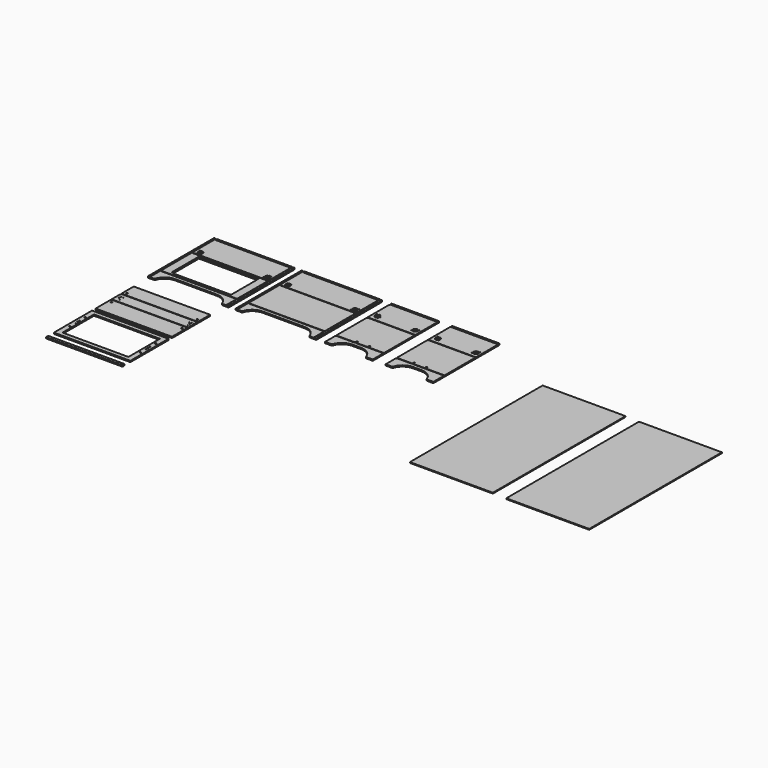
from build123d import *

# Parameters (mm, degrees)
F0_W          = 546.8
F0_H          = 275
F0_W_2        = 10
F0_H_2        = 600
F0_H_3        = 110.9
F0_H_4        = 76
F0_H_5        = 9.1
F0_H_6        = 10
F1_DEPTH      = 9
F0_W_3        = 435
F0_H_7        = 250.55
F0_W_4        = 425
F0_H_8        = 240.55
F0_W_5        = 185
F0_H_9        = 50
F0_W_6        = 345
F0_W_7        = 9.1
F0_H_10       = 17.1
F0_W_8        = 552.8
F0_H_11       = 345
F0_W_9        = 476.8
F0_H_12       = 285
F0_H_13       = 135.9
F0_H_14       = 80
F0_R          = 27.2912012127
F0_H_15       = 20
F2_DEPTH      = 3
F3_R          = 3.3
F3_R_2        = 17.5
F3_R_3        = 6
F3_R_4        = 5
F3_R_5        = 4.25
F3_R_6        = 2.5
F3_R_7        = 1.5
F4_DEPTH      = 16.75
F5_W          = 600
F5_H          = 1200
F6_DEPTH      = 6
F7_T1_DEPTH   = 9
F7_2_T1_DEPTH = 9
F7_3_T1_DEPTH = 9
F7_4_T1_DEPTH = 9
F8_R          = 5
F8_2_R        = 5
F8_3_R        = 5
F8_4_R        = 5


# Not quite as in the source:
# - a fillet or chamfer that OpenCascade refuses, or shapes differently, is made with other operations: its cross-section is extruded or revolved along the edge and cut away or added
# - a feature names something its author has since deleted; it is built from what else it names


with BuildPart() as f1:
    # F0 (on Top) → F1 (new body)
    with BuildSketch(Plane.XY):
        with Locations((752.7211838829, 673.5545394897)):
            Rectangle(F0_W, F0_H)
        with Locations((1040.2211838829, 735.2545394897)):
            Rectangle(F0_W_2, F0_H_2)
        with Locations((752.7211838829, 960.7045394897)):
            Rectangle(F0_W, F0_H_3)
        with Locations((752.7211838829, 858.1545394897)):
            Rectangle(F0_W, F0_H_4)
        Polygon((479.3211838829, 526.9545394897), (479.3211838829, 435.2545394897), (510.2211838829, 435.2545394897), (510.2211838829, 505.5045394897), (995.2211838829, 505.5045394897), (995.2211838829, 435.2545394897), (1026.1211838829, 435.2545394897), (1026.1211838829, 526.9545394897), align=None)
        with Locations((752.7211838829, 531.5045394897)):
            Rectangle(F0_W, F0_H_5)
        with Locations((465.2211838829, 735.2545394897)):
            Rectangle(F0_W_2, F0_H_2)
        with Locations((752.7211838829, 900.7045394897)):
            Rectangle(F0_W, F0_H_5)
        with Locations((752.7211838829, 815.6045394897)):
            Rectangle(F0_W, F0_H_5)
        Polygon((479.3211838829, 1035.2545394897), (470.2211838829, 1035.2545394897), (470.2211838829, 435.2545394897), (479.3211838829, 435.2545394897), (479.3211838829, 526.9545394897), (479.3211838829, 536.0545394897), (479.3211838829, 811.0545394897), (479.3211838829, 820.1545394897), (479.3211838829, 896.1545394897), (479.3211838829, 905.2545394897), (479.3211838829, 1016.1545394897), (479.3211838829, 1025.2545394897), align=None)
        Polygon((1035.2211838829, 1035.2545394897), (1026.1211838829, 1035.2545394897), (1026.1211838829, 1025.2545394897), (1026.1211838829, 1016.1545394897), (1026.1211838829, 905.2545394897), (1026.1211838829, 896.1545394897), (1026.1211838829, 820.1545394897), (1026.1211838829, 811.0545394897), (1026.1211838829, 536.0545394897), (1026.1211838829, 526.9545394897), (1026.1211838829, 435.2545394897), (1035.2211838829, 435.2545394897), align=None)
        with Locations((752.7211838829, 1030.2545394897)):
            Rectangle(F0_W, F0_H_6)
        with Locations((752.7211838829, 1020.7045394897)):
            Rectangle(F0_W, F0_H_5)
    extrude(amount=-F1_DEPTH)


with BuildPart() as f1b:
    # F0 (on Top) → F1, piece 2 (new body)
    with BuildSketch(Plane.XY):
        with Locations((118.6686661243, 673.5545394897)):
            Rectangle(F0_W, F0_H)
        with Locations((118.6686661243, 677.7795394897)):
            Rectangle(F0_W_3, F0_H_7, mode=Mode.SUBTRACT)
        with Locations((118.6686661243, 677.7795394897)):
            Rectangle(F0_W_3, F0_H_7)
        with Locations((118.6686661243, 677.7795394897)):
            Rectangle(F0_W_4, F0_H_8, mode=Mode.SUBTRACT)
        with Locations((118.6686661243, 960.7045394897)):
            Rectangle(F0_W, F0_H_3)
        with Locations((118.6686661243, 858.1545394897)):
            Rectangle(F0_W, F0_H_4)
        with Locations((118.6686661243, 851.8676246917)):
            Rectangle(F0_W_5, F0_H_9, mode=Mode.SUBTRACT)
        Polygon((-154.7313338757, 435.2545394897), (-123.8313338757, 435.2545394897), (-123.8313338757, 505.5045394897), (361.1686661243, 505.5045394897), (361.1686661243, 435.2545394897), (392.0686661243, 435.2545394897), (392.0686661243, 526.9545394897), (-154.7313338757, 526.9545394897), align=None)
        with Locations((118.6686661243, 851.8676246917)):
            Rectangle(F0_W_5, F0_H_9)
        with Locations((-168.8313338757, 735.2545394897)):
            Rectangle(F0_W_2, F0_H_2)
        with Locations((406.1686661243, 735.2545394897)):
            Rectangle(F0_W_2, F0_H_2)
        with Locations((118.6686661243, 1030.2545394897)):
            Rectangle(F0_W, F0_H_6)
        Polygon((-163.8313338757, 435.2545394897), (-154.7313338757, 435.2545394897), (-154.7313338757, 526.9545394897), (-154.7313338757, 536.0545394897), (-154.7313338757, 811.0545394897), (-154.7313338757, 820.1545394897), (-154.7313338757, 896.1545394897), (-154.7313338757, 905.2545394897), (-154.7313338757, 1016.1545394897), (-154.7313338757, 1025.2545394897), (-154.7313338757, 1035.2545394897), (-163.8313338757, 1035.2545394897), align=None)
        Polygon((392.0686661243, 536.0545394897), (392.0686661243, 526.9545394897), (392.0686661243, 435.2545394897), (401.1686661243, 435.2545394897), (401.1686661243, 1035.2545394897), (392.0686661243, 1035.2545394897), (392.0686661243, 1025.2545394897), (392.0686661243, 1016.1545394897), (392.0686661243, 905.2545394897), (392.0686661243, 896.1545394897), (392.0686661243, 820.1545394897), (392.0686661243, 811.0545394897), align=None)
        with Locations((118.6686661243, 900.7045394897)):
            Rectangle(F0_W, F0_H_5)
        with Locations((118.6686661243, 531.5045394897)):
            Rectangle(F0_W, F0_H_5)
        with Locations((118.6686661243, 1020.7045394897)):
            Rectangle(F0_W, F0_H_5)
        with Locations((118.6686661243, 815.6045394897)):
            Rectangle(F0_W, F0_H_5)
    extrude(amount=-F1_DEPTH)


with BuildPart() as f1c:
    # F0 (on Top) → F1, piece 3 (new body)
    with BuildSketch(Plane.XY):
        with Locations((1281.6600322723, 858.1545394897)):
            Rectangle(F0_W_6, F0_H_4)
        Polygon((1454.1600322723, 526.9545394897), (1109.1600322723, 526.9545394897), (1109.1600322723, 435.2545394897), (1159.1600322723, 435.2545394897), (1159.1600322723, 505.5045394897), (1404.1600322723, 505.5045394897), (1404.1600322723, 435.2545394897), (1454.1600322723, 435.2545394897), align=None)
        with Locations((1281.6600322723, 1030.2545394897)):
            Rectangle(F0_W_6, F0_H_6)
        Polygon((1454.1600322723, 811.0545394897), (1109.1600322723, 811.0545394897), (1109.1600322723, 536.0545394897), (1245.0600322723, 536.0545394897), (1245.0600322723, 553.1545394897), (1254.1600322723, 553.1545394897), (1254.1600322723, 536.0545394897), (1334.1600322723, 536.0545394897), (1334.1600322723, 553.1545394897), (1343.2600322723, 553.1545394897), (1343.2600322723, 536.0545394897), (1454.1600322723, 536.0545394897), align=None)
        with Locations((1281.6600322723, 815.6045394897)):
            Rectangle(F0_W_6, F0_H_5)
        with Locations((1281.6600322723, 900.7045394897)):
            Rectangle(F0_W_6, F0_H_5)
        Polygon((1245.0600322723, 536.0545394897), (1109.1600322723, 536.0545394897), (1109.1600322723, 526.9545394897), (1454.1600322723, 526.9545394897), (1454.1600322723, 536.0545394897), (1343.2600322723, 536.0545394897), (1334.1600322723, 536.0545394897), (1254.1600322723, 536.0545394897), align=None)
        with Locations((1281.6600322723, 1020.7045394897)):
            Rectangle(F0_W_6, F0_H_5)
        with Locations((1281.6600322723, 960.7045394897)):
            Rectangle(F0_W_6, F0_H_3)
        with Locations((1249.6100322723, 544.6045394897)):
            Rectangle(F0_W_7, F0_H_10)
        with Locations((1338.7100322723, 544.6045394897)):
            Rectangle(F0_W_7, F0_H_10)
    extrude(amount=-F1_DEPTH)


with BuildPart() as f1d:
    # F0 (on Top) → F1, piece 4 (new body)
    with BuildSketch(Plane.XY):
        with Locations((118.6686661243, -260.7726354599)):
            Rectangle(F0_W_8, F0_H_11)
        with Locations((118.6686661243, -260.7726354599)):
            Rectangle(F0_W_9, F0_H_12, mode=Mode.SUBTRACT)
    extrude(amount=-F1_DEPTH)


with BuildPart() as f1e:
    # F0 (on Top) → F1, piece 5 (new body)
    with BuildSketch(Plane.XY):
        with Locations((118.6686661243, 11.3700108051)):
            Rectangle(F0_W_8, F0_H_13)
        with Locations((118.6686661243, 232.9700108051)):
            Rectangle(F0_W_8, F0_H_3)
        with Locations((118.6686661243, 128.4200108051)):
            Rectangle(F0_W_8, F0_H_14)
        with Locations((132.2686661243, 128.4200108051)):
            Circle(F0_R, mode=Mode.SUBTRACT)
        with Locations((118.6686661243, 83.8700108051)):
            Rectangle(F0_W_8, F0_H_5)
        with Locations((118.6686661243, 172.9700108051)):
            Rectangle(F0_W_8, F0_H_5)
        with Locations((132.2686661243, 128.4200108051)):
            Circle(F0_R)
    extrude(amount=-F1_DEPTH)


with BuildPart() as f1f:
    # F0 (on Top) → F1, piece 6 (new body)
    with BuildSketch(Plane.XY):
        with Locations((118.6686661243, -494.1860234737)):
            Rectangle(F0_W_8, F0_H_15)
    extrude(amount=-F1_DEPTH)


with BuildPart() as f1g:
    # F0 (on Top) → F1, piece 7 (new body)
    with BuildSketch(Plane.XY):
        Polygon((1892.5400686264, 811.0545394897), (1547.5400686264, 811.0545394897), (1547.5400686264, 536.0545394897), (1658.4400686264, 536.0545394897), (1658.4400686264, 553.1545394897), (1667.5400686264, 553.1545394897), (1667.5400686264, 536.0545394897), (1747.5400686264, 536.0545394897), (1747.5400686264, 553.1545394897), (1756.6400686264, 553.1545394897), (1756.6400686264, 536.0545394897), (1892.5400686264, 536.0545394897), align=None)
        Polygon((1892.5400686264, 526.9545394897), (1547.5400686264, 526.9545394897), (1547.5400686264, 435.2545394897), (1597.5400686264, 435.2545394897), (1597.5400686264, 505.5045394897), (1842.5400686264, 505.5045394897), (1842.5400686264, 435.2545394897), (1892.5400686264, 435.2545394897), align=None)
        with Locations((1720.0400686264, 1030.2545394897)):
            Rectangle(F0_W_6, F0_H_6)
        with Locations((1720.0400686264, 858.1545394897)):
            Rectangle(F0_W_6, F0_H_4)
        with Locations((1720.0400686264, 960.7045394897)):
            Rectangle(F0_W_6, F0_H_3)
        with Locations((1720.0400686264, 815.6045394897)):
            Rectangle(F0_W_6, F0_H_5)
        Polygon((1658.4400686264, 536.0545394897), (1547.5400686264, 536.0545394897), (1547.5400686264, 526.9545394897), (1892.5400686264, 526.9545394897), (1892.5400686264, 536.0545394897), (1756.6400686264, 536.0545394897), (1747.5400686264, 536.0545394897), (1667.5400686264, 536.0545394897), align=None)
        with Locations((1720.0400686264, 1020.7045394897)):
            Rectangle(F0_W_6, F0_H_5)
        with Locations((1720.0400686264, 900.7045394897)):
            Rectangle(F0_W_6, F0_H_5)
        with Locations((1662.9900686264, 544.6045394897)):
            Rectangle(F0_W_7, F0_H_10)
        with Locations((1752.0900686264, 544.6045394897)):
            Rectangle(F0_W_7, F0_H_10)
    extrude(amount=-F1_DEPTH)


with BuildPart() as f2_tool:
    # F0 (on Top) → F2 (new body)
    with BuildSketch(Plane.XY):
        with Locations((118.6686661243, 815.6045394897)):
            Rectangle(F0_W, F0_H_5)
        Polygon((-163.8313338757, 435.2545394897), (-154.7313338757, 435.2545394897), (-154.7313338757, 526.9545394897), (-154.7313338757, 536.0545394897), (-154.7313338757, 811.0545394897), (-154.7313338757, 820.1545394897), (-154.7313338757, 896.1545394897), (-154.7313338757, 905.2545394897), (-154.7313338757, 1016.1545394897), (-154.7313338757, 1025.2545394897), (-154.7313338757, 1035.2545394897), (-163.8313338757, 1035.2545394897), align=None)
        with Locations((118.6686661243, 531.5045394897)):
            Rectangle(F0_W, F0_H_5)
        Polygon((392.0686661243, 536.0545394897), (392.0686661243, 526.9545394897), (392.0686661243, 435.2545394897), (401.1686661243, 435.2545394897), (401.1686661243, 1035.2545394897), (392.0686661243, 1035.2545394897), (392.0686661243, 1025.2545394897), (392.0686661243, 1016.1545394897), (392.0686661243, 905.2545394897), (392.0686661243, 896.1545394897), (392.0686661243, 820.1545394897), (392.0686661243, 811.0545394897), align=None)
        Polygon((479.3211838829, 1035.2545394897), (470.2211838829, 1035.2545394897), (470.2211838829, 435.2545394897), (479.3211838829, 435.2545394897), (479.3211838829, 526.9545394897), (479.3211838829, 536.0545394897), (479.3211838829, 811.0545394897), (479.3211838829, 820.1545394897), (479.3211838829, 896.1545394897), (479.3211838829, 905.2545394897), (479.3211838829, 1016.1545394897), (479.3211838829, 1025.2545394897), align=None)
        with Locations((752.7211838829, 815.6045394897)):
            Rectangle(F0_W, F0_H_5)
        with Locations((752.7211838829, 531.5045394897)):
            Rectangle(F0_W, F0_H_5)
        Polygon((1035.2211838829, 1035.2545394897), (1026.1211838829, 1035.2545394897), (1026.1211838829, 1025.2545394897), (1026.1211838829, 1016.1545394897), (1026.1211838829, 905.2545394897), (1026.1211838829, 896.1545394897), (1026.1211838829, 820.1545394897), (1026.1211838829, 811.0545394897), (1026.1211838829, 536.0545394897), (1026.1211838829, 526.9545394897), (1026.1211838829, 435.2545394897), (1035.2211838829, 435.2545394897), align=None)
        with Locations((1281.6600322723, 815.6045394897)):
            Rectangle(F0_W_6, F0_H_5)
        Polygon((1245.0600322723, 536.0545394897), (1109.1600322723, 536.0545394897), (1109.1600322723, 526.9545394897), (1454.1600322723, 526.9545394897), (1454.1600322723, 536.0545394897), (1343.2600322723, 536.0545394897), (1334.1600322723, 536.0545394897), (1254.1600322723, 536.0545394897), align=None)
        with Locations((118.6686661243, 1020.7045394897)):
            Rectangle(F0_W, F0_H_5)
        with Locations((752.7211838829, 1020.7045394897)):
            Rectangle(F0_W, F0_H_5)
        with Locations((1281.6600322723, 1020.7045394897)):
            Rectangle(F0_W_6, F0_H_5)
        with Locations((118.6686661243, 677.7795394897)):
            Rectangle(F0_W_3, F0_H_7)
        with Locations((118.6686661243, 677.7795394897)):
            Rectangle(F0_W_4, F0_H_8, mode=Mode.SUBTRACT)
        with Locations((118.6686661243, 172.9700108051)):
            Rectangle(F0_W_8, F0_H_5)
        with Locations((118.6686661243, 83.8700108051)):
            Rectangle(F0_W_8, F0_H_5)
        with Locations((1249.6100322723, 544.6045394897)):
            Rectangle(F0_W_7, F0_H_10)
        with Locations((1338.7100322723, 544.6045394897)):
            Rectangle(F0_W_7, F0_H_10)
        Polygon((1658.4400686264, 536.0545394897), (1547.5400686264, 536.0545394897), (1547.5400686264, 526.9545394897), (1892.5400686264, 526.9545394897), (1892.5400686264, 536.0545394897), (1756.6400686264, 536.0545394897), (1747.5400686264, 536.0545394897), (1667.5400686264, 536.0545394897), align=None)
        with Locations((1662.9900686264, 544.6045394897)):
            Rectangle(F0_W_7, F0_H_10)
        with Locations((1752.0900686264, 544.6045394897)):
            Rectangle(F0_W_7, F0_H_10)
        with Locations((1720.0400686264, 815.6045394897)):
            Rectangle(F0_W_6, F0_H_5)
        with Locations((1720.0400686264, 1020.7045394897)):
            Rectangle(F0_W_6, F0_H_5)
    extrude(amount=-F2_DEPTH)


with BuildPart() as f1_1:
    add(f1.part)

    # F2: cut by f2_tool
    add(f2_tool.part, mode=Mode.SUBTRACT)


with BuildPart() as f1b_1:
    add(f1b.part)

    # F2: cut by f2_tool
    add(f2_tool.part, mode=Mode.SUBTRACT)


with BuildPart() as f1c_1:
    add(f1c.part)

    # F2: cut by f2_tool
    add(f2_tool.part, mode=Mode.SUBTRACT)


with BuildPart() as f1e_1:
    add(f1e.part)

    # F2: cut by f2_tool
    add(f2_tool.part, mode=Mode.SUBTRACT)


with BuildPart() as f1g_1:
    add(f1g.part)

    # F2: cut by f2_tool
    add(f2_tool.part, mode=Mode.SUBTRACT)


with BuildPart() as f4_tool:
    # F3 (on Top) → F4 (new body)
    with BuildSketch(Plane.XY):
        with Locations((-138.6412364524, 865.0644420664)):
            Circle(F3_R)
        with Locations((-106.821431299, 833.244636913)):
            Circle(F3_R)
        with Locations((344.1587635476, 833.244636913)):
            Circle(F3_R)
        with Locations((375.978568701, 865.0644420664)):
            Circle(F3_R)
        with Locations((1160.069934849, 848.244636913)):
            Circle(F3_R)
        with Locations((1128.2501296956, 880.0644420664)):
            Circle(F3_R)
        with Locations((1435.069934849, 880.0644420664)):
            Circle(F3_R)
        with Locations((1403.2501296956, 848.244636913)):
            Circle(F3_R)
        with Locations((495.4112813062, 865.0644420664)):
            Circle(F3_R)
        with Locations((527.2310864596, 833.244636913)):
            Circle(F3_R)
        with Locations((1010.0310864596, 865.0644420664)):
            Circle(F3_R)
        with Locations((978.2112813062, 833.244636913)):
            Circle(F3_R)
        with Locations((-122.7313338757, 849.1545394897)):
            Circle(F3_R_2)
        with Locations((-122.7313338757, 849.1545394897)):
            Circle(F3_R_3, mode=Mode.SUBTRACT)
        with Locations((360.0686661243, 849.1545394897)):
            Circle(F3_R_2)
        with Locations((360.0686661243, 849.1545394897)):
            Circle(F3_R_3, mode=Mode.SUBTRACT)
        with Locations((511.3211838829, 849.1545394897)):
            Circle(F3_R_2)
        with Locations((511.3211838829, 849.1545394897)):
            Circle(F3_R_3, mode=Mode.SUBTRACT)
        with Locations((994.1211838829, 849.1545394897)):
            Circle(F3_R_2)
        with Locations((994.1211838829, 849.1545394897)):
            Circle(F3_R_3, mode=Mode.SUBTRACT)
        with Locations((1144.1600322723, 864.1545394897)):
            Circle(F3_R_2)
        with Locations((1144.1600322723, 864.1545394897)):
            Circle(F3_R_3, mode=Mode.SUBTRACT)
        with Locations((1419.1600322723, 864.1545394897)):
            Circle(F3_R_2)
        with Locations((1419.1600322723, 864.1545394897)):
            Circle(F3_R_3, mode=Mode.SUBTRACT)
        with Locations((-134.7313338757, 198.4200108051)):
            Circle(F3_R_4)
        with Locations((-134.7313338757, 58.4200108051)):
            Circle(F3_R_4)
        with Locations((375.0686661243, 198.4200108051)):
            Circle(F3_R_4)
        with Locations((375.0686661243, 58.4200108051)):
            Circle(F3_R_4)
        with Locations((-134.7313338757, -178.2726354599)):
            Circle(F3_R_4)
        with Locations((-134.7313338757, -318.2726354599)):
            Circle(F3_R_4)
        with Locations((375.0686661243, -178.2726354599)):
            Circle(F3_R_4)
        with Locations((375.0686661243, -318.2726354599)):
            Circle(F3_R_4)
        with Locations((-134.7313338757, 128.4200108051)):
            Circle(F3_R_5)
        with Locations((375.0686661243, 128.4200108051)):
            Circle(F3_R_5)
        with Locations((375.0686661243, -248.2726354599)):
            Circle(F3_R_5)
        with Locations((-134.7313338757, -248.2726354599)):
            Circle(F3_R_5)
        with Locations((-134.7313338757, -230.0226354599)):
            Circle(F3_R_6)
        with Locations((-134.7313338757, -266.5226354599)):
            Circle(F3_R_6)
        with Locations((375.0686661243, -230.0226354599)):
            Circle(F3_R_6)
        with Locations((375.0686661243, -266.5226354599)):
            Circle(F3_R_6)
        with Locations((375.0686661243, 146.6700108051)):
            Circle(F3_R_6)
        with Locations((375.0686661243, 110.1700108051)):
            Circle(F3_R_6)
        with Locations((-134.7313338757, 146.6700108051)):
            Circle(F3_R_6)
        with Locations((-134.7313338757, 110.1700108051)):
            Circle(F3_R_6)
        with Locations((-413.0307251624, 651.5564784469)):
            Circle(F3_R_7)
        with Locations((-382.0594481464, 651.5564784469)):
            Circle(F3_R_7)
        with Locations((-382.0594481464, 620.5852014309)):
            Circle(F3_R_7)
        with Locations((-413.0307251624, 620.5852014309)):
            Circle(F3_R_7)
        with Locations((360.0686661243, 871.0545394897)):
            Circle(F3_R_7)
        with Locations((381.9686661243, 849.1545394897)):
            Circle(F3_R_7)
        with Locations((360.0686661243, 827.2545394897)):
            Circle(F3_R_7)
        with Locations((338.1686661243, 849.1545394897)):
            Circle(F3_R_7)
        with Locations((1144.1600322723, 886.0545394897)):
            Circle(F3_R_7)
        with Locations((1166.0600322723, 864.1545394897)):
            Circle(F3_R_7)
        with Locations((1144.1600322723, 842.2545394897)):
            Circle(F3_R_7)
        with Locations((1122.2600322723, 864.1545394897)):
            Circle(F3_R_7)
        with Locations((-150.2169723836, 143.9056493131)):
            Circle(F3_R_7)
        with Locations((-119.2456953677, 143.9056493131)):
            Circle(F3_R_7)
        with Locations((-119.2456953677, 112.9343722971)):
            Circle(F3_R_7)
        with Locations((-150.2169723836, 112.9343722971)):
            Circle(F3_R_7)
        with Locations((359.5830276164, 143.9056493131)):
            Circle(F3_R_7)
        with Locations((390.5543046323, 143.9056493131)):
            Circle(F3_R_7)
        with Locations((390.5543046323, 112.9343722971)):
            Circle(F3_R_7)
        with Locations((359.5830276164, 112.9343722971)):
            Circle(F3_R_7)
        with Locations((1873.4499712031, 880.0644420664)):
            Circle(F3_R)
        with Locations((1841.6301660497, 848.244636913)):
            Circle(F3_R)
        with Locations((1857.5400686264, 864.1545394897)):
            Circle(F3_R_2)
        with Locations((1857.5400686264, 864.1545394897)):
            Circle(F3_R_3, mode=Mode.SUBTRACT)
        with Locations((1566.6301660497, 880.0644420664)):
            Circle(F3_R)
        with Locations((1598.4499712031, 848.244636913)):
            Circle(F3_R)
        with Locations((1582.5400686264, 864.1545394897)):
            Circle(F3_R_2)
        with Locations((1582.5400686264, 864.1545394897)):
            Circle(F3_R_3, mode=Mode.SUBTRACT)
        with Locations((-122.7313338757, 849.1545394897)):
            Circle(F3_R_3)
        with Locations((360.0686661243, 849.1545394897)):
            Circle(F3_R_3)
        with Locations((511.3211838829, 849.1545394897)):
            Circle(F3_R_3)
        with Locations((994.1211838829, 849.1545394897)):
            Circle(F3_R_3)
        with Locations((1419.1600322723, 864.1545394897)):
            Circle(F3_R_3)
        with Locations((1144.1600322723, 864.1545394897)):
            Circle(F3_R_3)
        with Locations((1582.5400686264, 864.1545394897)):
            Circle(F3_R_3)
        with Locations((1857.5400686264, 864.1545394897)):
            Circle(F3_R_3)
    extrude(amount=-F4_DEPTH)


with BuildPart() as f1_2:
    add(f1_1.part)

    # F4: cut by f4_tool
    add(f4_tool.part, mode=Mode.SUBTRACT)

    # F7: fillet of radius 94.7578823231 on 2 edges, made by hand

    # F7_s2 → F7_t1 (join)
    with BuildSketch(Plane.XY.offset(-9)):
        with BuildLine():
            ThreePointArc((510.2211838829, 435.2545394897), (544.0628608142, 485.9176997679), (601.7548933369, 505.5045394897))
            Line((601.7548933369, 505.5045394897), (510.2211838829, 505.5045394897))
            Line((510.2211838829, 505.5045394897), (510.2211838829, 435.2545394897))
        make_face()
        with BuildLine():
            ThreePointArc((903.6874744289, 505.5045394897), (961.3795069516, 485.9176997679), (995.2211838829, 435.2545394897))
            Line((995.2211838829, 435.2545394897), (995.2211838829, 505.5045394897))
            Line((995.2211838829, 505.5045394897), (903.6874744289, 505.5045394897))
        make_face()
    extrude(amount=F7_T1_DEPTH)

    # F8
    f8_edges = [f1_2.edges().sort_by_distance(p)[0] for p in [
        (460.221184, 1035.254539, -4.5),
        (1045.221184, 1035.254539, -4.5),
        (1045.221184, 435.254539, -4.5),
        (460.221184, 435.254539, -4.5),
        (510.221184, 435.254539, -4.5),
        (995.221184, 435.254539, -4.5),
    ]]
    fillet(f8_edges, radius=F8_R)


with BuildPart() as f1b_2:
    add(f1b_1.part)

    # F4: cut by f4_tool
    add(f4_tool.part, mode=Mode.SUBTRACT)

    # F7#2: fillet of radius 94.7578823231 on 2 edges, made by hand

    # F7_2_s2 → F7_2_t1 (join)
    with BuildSketch(Plane.XY.offset(-9)):
        with BuildLine():
            ThreePointArc((-123.8313338757, 435.2545394897), (-89.9896569444, 485.9176997679), (-32.2976244217, 505.5045394897))
            Line((-32.2976244217, 505.5045394897), (-123.8313338757, 505.5045394897))
            Line((-123.8313338757, 505.5045394897), (-123.8313338757, 435.2545394897))
        make_face()
        with BuildLine():
            ThreePointArc((269.6349566704, 505.5045394897), (327.3269891931, 485.9176997679), (361.1686661243, 435.2545394897))
            Line((361.1686661243, 435.2545394897), (361.1686661243, 505.5045394897))
            Line((361.1686661243, 505.5045394897), (269.6349566704, 505.5045394897))
        make_face()
    extrude(amount=F7_2_T1_DEPTH)

    # F8#2
    f8_2_edges = [f1b_2.edges().sort_by_distance(p)[0] for p in [
        (-173.831334, 1035.254539, -4.5),
        (411.168666, 1035.254539, -4.5),
        (411.168666, 435.254539, -4.5),
        (-173.831334, 435.254539, -4.5),
        (-123.831334, 435.254539, -4.5),
        (361.168666, 435.254539, -4.5),
    ]]
    fillet(f8_2_edges, radius=F8_2_R)


with BuildPart() as f1c_2:
    add(f1c_1.part)

    # F4: cut by f4_tool
    add(f4_tool.part, mode=Mode.SUBTRACT)

    # F7#3: fillet of radius 94.7578823231 on 2 edges, made by hand

    # F7_3_s2 → F7_3_t1 (join)
    with BuildSketch(Plane.XY.offset(-9)):
        with BuildLine():
            ThreePointArc((1159.1600322723, 435.2545394897), (1193.0017092036, 485.9176997679), (1250.6937417263, 505.5045394897))
            Line((1250.6937417263, 505.5045394897), (1159.1600322723, 505.5045394897))
            Line((1159.1600322723, 505.5045394897), (1159.1600322723, 435.2545394897))
        make_face()
        with BuildLine():
            ThreePointArc((1312.6263228184, 505.5045394897), (1370.3183553411, 485.9176997679), (1404.1600322723, 435.2545394897))
            Line((1404.1600322723, 435.2545394897), (1404.1600322723, 505.5045394897))
            Line((1404.1600322723, 505.5045394897), (1312.6263228184, 505.5045394897))
        make_face()
    extrude(amount=F7_3_T1_DEPTH)

    # F8#3
    f8_3_edges = [f1c_2.edges().sort_by_distance(p)[0] for p in [
        (1159.160032, 435.254539, -4.5),
        (1404.160032, 435.254539, -4.5),
    ]]
    fillet(f8_3_edges, radius=F8_3_R)


with BuildPart() as f1d_1:
    add(f1d.part)

    # F4: cut by f4_tool
    add(f4_tool.part, mode=Mode.SUBTRACT)


with BuildPart() as f1e_2:
    add(f1e_1.part)

    # F4: cut by f4_tool
    add(f4_tool.part, mode=Mode.SUBTRACT)


with BuildPart() as f1g_2:
    add(f1g_1.part)

    # F4: cut by f4_tool
    add(f4_tool.part, mode=Mode.SUBTRACT)

    # F7#4: fillet of radius 94.7578823231 on 2 edges, made by hand

    # F7_4_s2 → F7_4_t1 (join)
    with BuildSketch(Plane.XY.offset(-9)):
        with BuildLine():
            ThreePointArc((1597.5400686264, 435.2545394897), (1631.3817455577, 485.9176997679), (1689.0737780804, 505.5045394897))
            Line((1689.0737780804, 505.5045394897), (1597.5400686264, 505.5045394897))
            Line((1597.5400686264, 505.5045394897), (1597.5400686264, 435.2545394897))
        make_face()
        with BuildLine():
            ThreePointArc((1751.0063591724, 505.5045394897), (1808.6983916951, 485.9176997679), (1842.5400686264, 435.2545394897))
            Line((1842.5400686264, 435.2545394897), (1842.5400686264, 505.5045394897))
            Line((1842.5400686264, 505.5045394897), (1751.0063591724, 505.5045394897))
        make_face()
    extrude(amount=F7_4_T1_DEPTH)

    # F8#4
    f8_4_edges = [f1g_2.edges().sort_by_distance(p)[0] for p in [
        (1597.540069, 435.254539, -4.5),
        (1842.540069, 435.254539, -4.5),
    ]]
    fillet(f8_4_edges, radius=F8_4_R)


with BuildPart() as f6:
    # F5 (on Top) → F6 (new body)
    with BuildSketch(Plane.XY):
        with Locations((2709.5732895526, 176.8627604207)):
            Rectangle(F5_W, F5_H)
    extrude(amount=F6_DEPTH)


with BuildPart() as f6b:
    # F5 (on Top) → F6, piece 2 (new body)
    with BuildSketch(Plane.XY):
        with Locations((3411.2807133674, 171.2094245166)):
            Rectangle(F5_W, F5_H)
    extrude(amount=F6_DEPTH)


solid = Compound([f1f.part, f1_2.part, f1b_2.part, f1c_2.part, f1d_1.part, f1e_2.part, f1g_2.part, f6.part, f6b.part])
